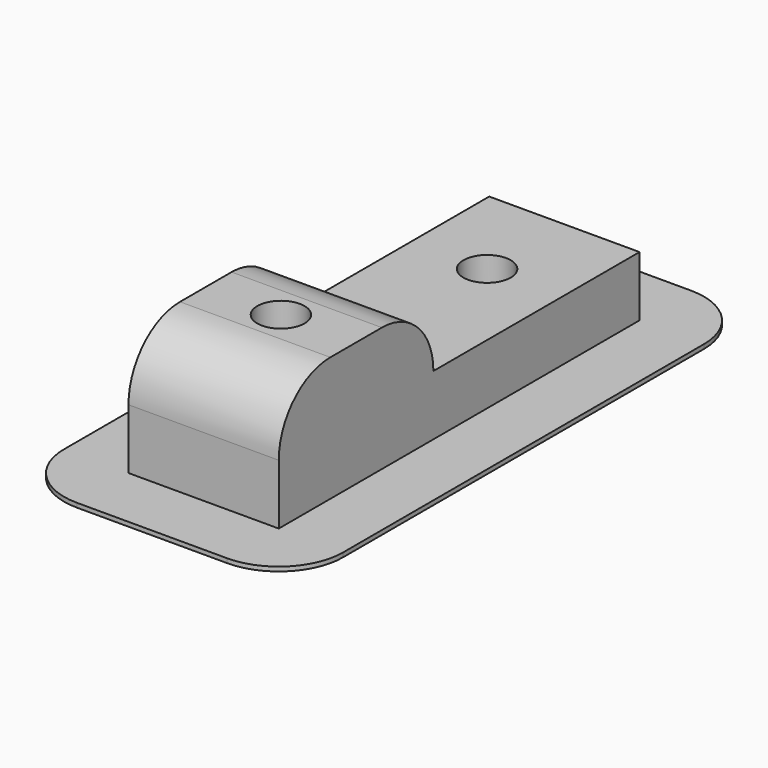
from build123d import *

# Parameters (mm, degrees)
F1_DEPTH = 7
F2_R     = 2.99999
F3_R     = 1.1
F4_DEPTH = 6.001
F5_W     = 7
F5_H     = 21
F6_DEPTH = 0.2


# Not quite as in the source:
# - a fillet or chamfer is up to 0.001 mm smaller than in the source, because OpenCascade refuses the exact size


with BuildPart() as f1:
    # F0 (on Right) → F1 (new body)
    with BuildSketch(Plane.YZ):
        Polygon((-21, 0), (0, 0), (0, 3), (-12, 3), (-12, 6), (-21, 6), align=None)
    extrude(amount=F1_DEPTH)

    # F2 (radius 3 in the source; OpenCascade refuses exactly that, so slightly less here)
    f2_edges = [f1.edges().sort_by_distance(p)[0] for p in [
        (3.5, -12, 6),
        (3.5, -21, 6),
    ]]
    fillet(f2_edges, radius=F2_R)

    # F3 (on face) → F4 (cut, through all)
    with BuildSketch(Plane(origin=(0, 0, 0), x_dir=(1, 0, 0), z_dir=(0, 0, -1))):
        with Locations((3.5, 16.5)):
            Circle(F3_R)
        with Locations((3.5, 4.5)):
            Circle(F3_R)
    extrude(amount=-F4_DEPTH, mode=Mode.SUBTRACT)

    # F5 (on face) → F6 (join)
    with BuildSketch(Plane(origin=(0, 0, 0), x_dir=(1, 0, 0), z_dir=(0, 0, -1))):
        with BuildLine():
            ThreePointArc((0, 24), (-2.1213203436, 23.1213203436), (-3, 21))
            Line((-3, 21), (-3, 0))
            ThreePointArc((-3, 0), (-2.1213203436, -2.1213203436), (0, -3))
            Line((0, -3), (7, -3))
            ThreePointArc((7, -3), (9.1213203436, -2.1213203436), (10, 0))
            Line((10, 0), (10, 21))
            ThreePointArc((10, 21), (9.1213203436, 23.1213203436), (7, 24))
            Line((7, 24), (0, 24))
        make_face()
        with Locations((3.5, 10.5)):
            Rectangle(F5_W, F5_H, mode=Mode.SUBTRACT)
    extrude(amount=-F6_DEPTH)


solid = f1.part
